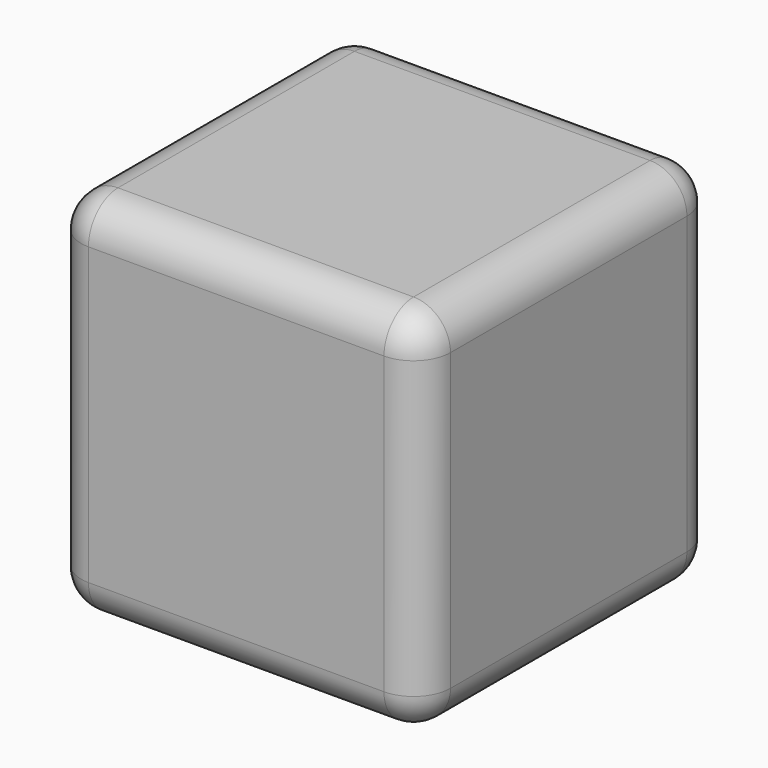
from build123d import *

# Parameters (mm, degrees)
F0_W     = 50.8
F0_H     = 50.8
F1_DEPTH = 50.8
F2_R     = 5.08
F3_T     = -2.54


# Not quite as in the source:
# - a shell that OpenCascade refuses in one call is made with other operations: the cavity is built on its own and cut out


with BuildPart() as f1:
    # F0 (on Top) → F1 (new body)
    with BuildSketch(Plane.XY):
        Rectangle(F0_W, F0_H)
    extrude(amount=F1_DEPTH)

    # F2
    f2_edges = [f1.edges().sort_by_distance(p)[0] for p in [
        (-25.4, 0, 0),
        (-25.4, 0, 50.8),
        (-25.4, 25.4, 25.4),
        (25.4, 0, 50.8),
        (0, 25.4, 50.8),
        (0, -25.4, 50.8),
        (-25.4, -25.4, 25.4),
        (25.4, 25.4, 25.4),
        (0, 25.4, 0),
        (25.4, 0, 0),
        (25.4, -25.4, 25.4),
        (0, -25.4, 0),
    ]]
    fillet(f2_edges, radius=F2_R)

    # F3: a shell. OpenCascade refuses it in one call, so the cavity is built on its own and cut out:
    # the body offset inwards by the wall thickness, plus a prism from it out through each open face.
    f3_core = offset(f1.part, amount=F3_T, mode=Mode.PRIVATE)
    f3_exits = [f3_core.faces().sort_by_distance(p)[0] for p in [
        (0, 0, 2.54),
    ]]
    add(f3_core, mode=Mode.SUBTRACT)
    extrude(f3_exits, amount=-F3_T, mode=Mode.SUBTRACT)


solid = f1.part
